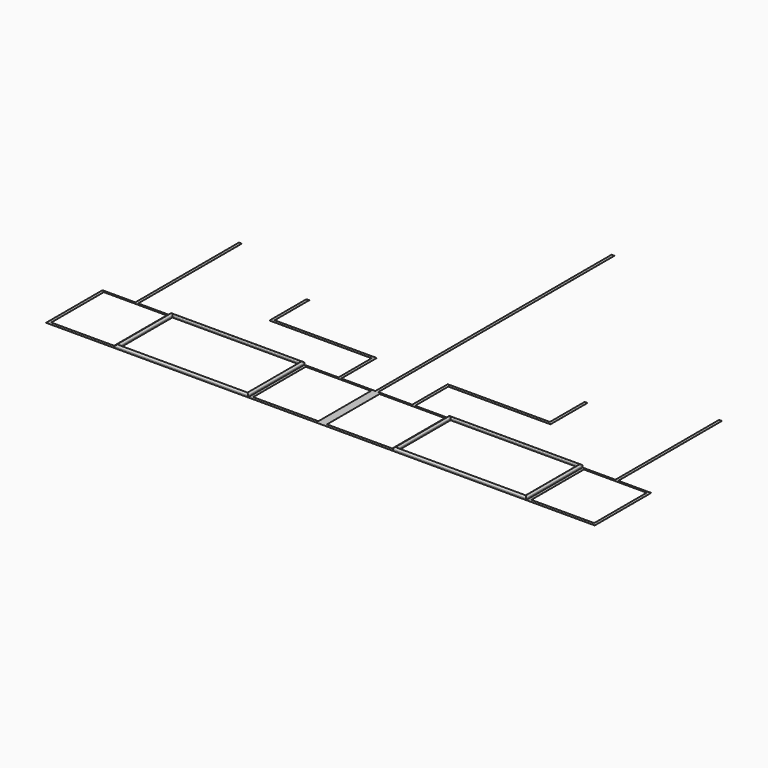
from build123d import *

# Parameters (mm, degrees)
F0_W         = 9.525
F0_H         = 457.2
F1_DEPTH     = 0.254
F0_W_2       = 19.05
F0_H_2       = 863.6
F2_DEPTH     = 19.05
F3_T1_DEPTH  = 936.625
F3_T3_DEPTH  = 517.525
F3_T5_DEPTH  = 850.9
F3_T7_DEPTH  = 438.15
F3_T13_DEPTH = 874.7125
F3_T17_DEPTH = 461.9625
F3_T24_DEPTH = 874.7125
F3_T28_DEPTH = 461.9625
F3_T35_DEPTH = 461.9625
F3_T39_DEPTH = 874.7125
F3_T46_DEPTH = 874.7125
F3_T50_DEPTH = 461.9625
F4_DEPTH     = 0.254
F5_DEPTH     = 19.05
F6_T3_DEPTH  = 517.525
F6_T6_DEPTH  = 936.625
F6_T9_DEPTH  = 517.525
F6_T12_DEPTH = 936.625
F6_T15_DEPTH = 850.9
F6_T18_DEPTH = 438.15
F6_T21_DEPTH = 850.9
F6_T24_DEPTH = 438.15
F6_T28_DEPTH = 874.7125
F6_T32_DEPTH = 461.9625
F6_T38_DEPTH = 874.7125
F6_T42_DEPTH = 461.9625
F6_T48_DEPTH = 461.9625
F6_T52_DEPTH = 874.7125
F6_T58_DEPTH = 874.7125
F6_T62_DEPTH = 461.9625


# Not quite as in the source:
# - a fillet or chamfer that OpenCascade refuses, or shapes differently, is made with other operations: its cross-section is extruded or revolved along the edge and cut away or added
# - a feature names something its author has since deleted; it is built from what else it names


with BuildPart() as f1:
    # F0 (on Top) → F1 (new body)
    with BuildSketch(Plane.XY):
        Polygon((0, -793.75), (0, 1187.45), (-9.525, 1187.45), (-9.525, -781.05), (-9.525, -793.75), align=None)
        with Locations((-4.7625, -1022.35)):
            Rectangle(F0_W, F0_H)
        Polygon((-9.525, -793.75), (-9.525, -781.05), (-28.575, -781.05), (-236.5375, -781.05), (-255.5875, -781.05), (-463.55, -781.05), (-482.6, -781.05), (-482.6, -793.75), (-482.6, -1250.95), (-9.525, -1250.95), align=None)
        Polygon((-28.575, -1231.9), (-463.55, -1231.9), (-463.55, -793.75), (-255.5875, -793.75), (-236.5375, -793.75), (-28.575, -793.75), align=None, mode=Mode.SUBTRACT)
        Polygon((-255.5875, -781.05), (-236.5375, -781.05), (-236.5375, -485.775), (-917.575, -485.775), (-917.575, -196.85), (-936.625, -196.85), (-936.625, -504.825), (-936.3493996177, -504.825), (-917.575, -504.825), (-255.5875, -504.825), align=None)
    extrude(amount=F1_DEPTH)

    # F0 (on Top) → F4 (join)
    with BuildSketch(Plane.XY):
        Polygon((9.525, -781.05), (9.525, -793.75), (9.525, -1250.95), (482.6, -1250.95), (482.6, -793.75), (482.6, -781.05), (463.55, -781.05), (255.5875, -781.05), (236.5375, -781.05), (28.575, -781.05), align=None)
        Polygon((28.575, -793.75), (236.5375, -793.75), (255.5875, -793.75), (463.55, -793.75), (463.55, -1231.9), (28.575, -1231.9), align=None, mode=Mode.SUBTRACT)
        with Locations((4.7625, -1022.35)):
            Rectangle(F0_W, F0_H)
        with Locations((-4.7625, -1022.35)):
            Rectangle(F0_W, F0_H)
        Polygon((0, -793.75), (0, 1187.45), (-9.525, 1187.45), (-9.525, -781.05), (-9.525, -793.75), align=None)
        Polygon((9.525, 1187.45), (0, 1187.45), (0, -793.75), (9.525, -793.75), (9.525, -781.05), align=None)
        Polygon((236.5375, -485.775), (236.5375, -781.05), (255.5875, -781.05), (255.5875, -504.825), (917.575, -504.825), (936.3493996177, -504.825), (936.625, -504.825), (936.625, -196.85), (917.575, -196.85), (917.575, -485.775), align=None)
    extrude(amount=F4_DEPTH)


with BuildPart() as f1b:
    # F0 (on Top) → F1, piece 2 (new body)
    with BuildSketch(Plane.XY):
        Polygon((-1809.75, -781.05), (-1828.8, -781.05), (-1828.8, -1250.95), (-1371.6, -1250.95), (-1371.6, -793.75), (-1371.6, -781.05), (-1390.65, -781.05), (-1590.675, -781.05), (-1609.725, -781.05), align=None)
        Polygon((-1809.75, -1231.9), (-1809.75, -793.75), (-1609.725, -793.75), (-1590.675, -793.75), (-1390.65, -793.75), (-1390.65, -1231.9), align=None, mode=Mode.SUBTRACT)
        with Locations((-1600.2, -349.25)):
            Rectangle(F0_W_2, F0_H_2)
    extrude(amount=F1_DEPTH)


with BuildPart() as f2:
    # F0 (on Top) → F2 (new body)
    with BuildSketch(Plane.XY):
        Polygon((-1371.6, -1250.95), (-482.6, -1250.95), (-482.6, -793.75), (-482.6, -781.05), (-501.65, -781.05), (-1352.55, -781.05), (-1371.6, -781.05), (-1371.6, -793.75), align=None)
        Polygon((-501.65, -1231.9), (-1352.55, -1231.9), (-1352.55, -793.75), (-927.1, -793.75), (-501.65, -793.75), align=None, mode=Mode.SUBTRACT)
    extrude(amount=F2_DEPTH)

    # F3: fillet of radius 9.525 on 8 edges, made by hand

    # F3_s2 → F3_t1 (cut)
    with BuildSketch(Plane.YZ.offset(-1395.4125)):
        with BuildLine():
            ThreePointArc((-1250.95, 9.525), (-1248.1601920908, 16.2601920908), (-1241.425, 19.05))
            Line((-1241.425, 19.05), (-1250.95, 19.05))
            Line((-1250.95, 19.05), (-1250.95, 9.525))
        make_face()
        with BuildLine():
            ThreePointArc((-790.575, 19.05), (-783.8398079092, 16.2601920908), (-781.05, 9.525))
            Line((-781.05, 9.525), (-781.05, 19.05))
            Line((-781.05, 19.05), (-790.575, 19.05))
        make_face()
    extrude(amount=F3_T1_DEPTH, mode=Mode.SUBTRACT)

    # F3_s4 → F3_t3 (cut)
    with BuildSketch(Plane.XZ.offset(757.2375)):
        with BuildLine():
            ThreePointArc((-492.125, 19.05), (-485.3898079092, 16.2601920908), (-482.6, 9.525))
            Line((-482.6, 9.525), (-482.6, 19.05))
            Line((-482.6, 19.05), (-492.125, 19.05))
        make_face()
        with BuildLine():
            ThreePointArc((-1362.075, 19.05), (-1368.8101920908, 16.2601920908), (-1371.6, 9.525))
            Line((-1371.6, 9.525), (-1371.6, 19.05))
            Line((-1371.6, 19.05), (-1362.075, 19.05))
        make_face()
    extrude(amount=F3_T3_DEPTH, mode=Mode.SUBTRACT)

    # F3_s6 → F3_t5 (cut)
    with BuildSketch(Plane.YZ.offset(-1352.55)):
        with BuildLine():
            ThreePointArc((-1241.425, 19.05), (-1234.6898079092, 16.2601920908), (-1231.9, 9.525))
            Line((-1231.9, 9.525), (-1231.9, 19.05))
            Line((-1231.9, 19.05), (-1241.425, 19.05))
        make_face()
        with BuildLine():
            ThreePointArc((-784.225, 19.05), (-790.9601920908, 16.2601920908), (-793.75, 9.525))
            Line((-793.75, 9.525), (-793.75, 19.05))
            Line((-793.75, 19.05), (-784.225, 19.05))
        make_face()
    extrude(amount=F3_T5_DEPTH, mode=Mode.SUBTRACT)

    # F3_s8 → F3_t7 (cut)
    with BuildSketch(Plane.XZ.offset(793.75)):
        with BuildLine():
            ThreePointArc((-1362.075, 19.05), (-1355.3398079092, 16.2601920908), (-1352.55, 9.525))
            Line((-1352.55, 9.525), (-1352.55, 19.05))
            Line((-1352.55, 19.05), (-1362.075, 19.05))
        make_face()
        with BuildLine():
            ThreePointArc((-492.125, 19.05), (-498.8601920908, 16.2601920908), (-501.65, 9.525))
            Line((-501.65, 9.525), (-501.65, 19.05))
            Line((-501.65, 19.05), (-492.125, 19.05))
        make_face()
    extrude(amount=F3_T7_DEPTH, mode=Mode.SUBTRACT)


with BuildPart() as f3_tool11:
    # F3_s12 → F3_t13 (new body)
    with BuildSketch(Plane.YZ.offset(-477.8375)):
        with BuildLine():
            ThreePointArc((-1241.425, 19.05), (-1234.6898079092, 16.2601920908), (-1231.9, 9.525))
            Line((-1231.9, 9.525), (-1231.9, 19.05))
            Line((-1231.9, 19.05), (-1241.425, 19.05))
        make_face()
    extrude(amount=-F3_T13_DEPTH)

    split(bisect_by=Plane.YZ.offset(-501.65), keep=Keep.TOP)


with BuildPart() as f3_tool15:
    # F3_s16 → F3_t17 (new body)
    with BuildSketch(Plane.XZ.offset(793.75)):
        with BuildLine():
            ThreePointArc((-492.125, 19.05), (-498.8601920908, 16.2601920908), (-501.65, 9.525))
            Line((-501.65, 9.525), (-501.65, 19.05))
            Line((-501.65, 19.05), (-492.125, 19.05))
        make_face()
    extrude(amount=F3_T17_DEPTH)

    split(bisect_by=Plane.XZ.offset(1231.9), keep=Keep.TOP)


with BuildPart() as f3_tool11_1:
    add(f3_tool11.part)

    # F3_t19: intersect F3_tool15
    add(f3_tool15.part, mode=Mode.INTERSECT)


with BuildPart() as f2_1:
    add(f2.part)

    # F3_t9: cut F3_tool11
    add(f3_tool11_1.part, mode=Mode.SUBTRACT)


with BuildPart() as f3_tool22:
    # F3_s23 → F3_t24 (new body)
    with BuildSketch(Plane.YZ.offset(-501.65)):
        with BuildLine():
            ThreePointArc((-1241.425, 19.05), (-1234.6898079092, 16.2601920908), (-1231.9, 9.525))
            Line((-1231.9, 9.525), (-1231.9, 19.05))
            Line((-1231.9, 19.05), (-1241.425, 19.05))
        make_face()
    extrude(amount=-F3_T24_DEPTH)

    split(bisect_by=Plane.YZ.offset(-1352.55), keep=Keep.BOTTOM)


with BuildPart() as f3_tool26:
    # F3_s27 → F3_t28 (new body)
    with BuildSketch(Plane.XZ.offset(1255.7125)):
        with BuildLine():
            ThreePointArc((-1362.075, 19.05), (-1355.3398079092, 16.2601920908), (-1352.55, 9.525))
            Line((-1352.55, 9.525), (-1352.55, 19.05))
            Line((-1352.55, 19.05), (-1362.075, 19.05))
        make_face()
    extrude(amount=-F3_T28_DEPTH)

    split(bisect_by=Plane.XZ.offset(1231.9), keep=Keep.TOP)


with BuildPart() as f3_tool22_1:
    add(f3_tool22.part)

    # F3_t30: intersect F3_tool26
    add(f3_tool26.part, mode=Mode.INTERSECT)


with BuildPart() as f2_2:
    add(f2_1.part)

    # F3_t20: cut F3_tool22
    add(f3_tool22_1.part, mode=Mode.SUBTRACT)


with BuildPart() as f3_tool33:
    # F3_s34 → F3_t35 (new body)
    with BuildSketch(Plane.XZ.offset(1231.9)):
        with BuildLine():
            ThreePointArc((-1362.075, 19.05), (-1355.3398079092, 16.2601920908), (-1352.55, 9.525))
            Line((-1352.55, 9.525), (-1352.55, 19.05))
            Line((-1352.55, 19.05), (-1362.075, 19.05))
        make_face()
    extrude(amount=-F3_T35_DEPTH)

    split(bisect_by=Plane.XZ.offset(793.75), keep=Keep.BOTTOM)


with BuildPart() as f3_tool37:
    # F3_s38 → F3_t39 (new body)
    with BuildSketch(Plane.YZ.offset(-501.65)):
        with BuildLine():
            ThreePointArc((-784.225, 19.05), (-790.9601920908, 16.2601920908), (-793.75, 9.525))
            Line((-793.75, 9.525), (-793.75, 19.05))
            Line((-793.75, 19.05), (-784.225, 19.05))
        make_face()
    extrude(amount=-F3_T39_DEPTH)

    split(bisect_by=Plane.YZ.offset(-1352.55), keep=Keep.BOTTOM)


with BuildPart() as f3_tool33_1:
    add(f3_tool33.part)

    # F3_t41: intersect F3_tool37
    add(f3_tool37.part, mode=Mode.INTERSECT)


with BuildPart() as f2_3:
    add(f2_2.part)

    # F3_t31: cut F3_tool33
    add(f3_tool33_1.part, mode=Mode.SUBTRACT)


with BuildPart() as f3_tool44:
    # F3_s45 → F3_t46 (new body)
    with BuildSketch(Plane.YZ.offset(-477.8375)):
        with BuildLine():
            ThreePointArc((-784.225, 19.05), (-790.9601920908, 16.2601920908), (-793.75, 9.525))
            Line((-793.75, 9.525), (-793.75, 19.05))
            Line((-793.75, 19.05), (-784.225, 19.05))
        make_face()
    extrude(amount=-F3_T46_DEPTH)

    split(bisect_by=Plane.YZ.offset(-501.65), keep=Keep.TOP)


with BuildPart() as f3_tool48:
    # F3_s49 → F3_t50 (new body)
    with BuildSketch(Plane.XZ.offset(769.9375)):
        with BuildLine():
            ThreePointArc((-492.125, 19.05), (-498.8601920908, 16.2601920908), (-501.65, 9.525))
            Line((-501.65, 9.525), (-501.65, 19.05))
            Line((-501.65, 19.05), (-492.125, 19.05))
        make_face()
    extrude(amount=F3_T50_DEPTH)

    split(bisect_by=Plane.XZ.offset(793.75), keep=Keep.BOTTOM)


with BuildPart() as f3_tool44_1:
    add(f3_tool44.part)

    # F3_t52: intersect F3_tool48
    add(f3_tool48.part, mode=Mode.INTERSECT)


with BuildPart() as f2_4:
    add(f2_3.part)

    # F3_t42: cut F3_tool44
    add(f3_tool44_1.part, mode=Mode.SUBTRACT)


with BuildPart() as f4:
    # F0 (on Top) → F4, piece 2 (new body)
    with BuildSketch(Plane.XY):
        with Locations((1600.2, -349.25)):
            Rectangle(F0_W_2, F0_H_2)
        Polygon((1828.8, -1250.95), (1828.8, -781.05), (1809.75, -781.05), (1609.725, -781.05), (1590.675, -781.05), (1390.65, -781.05), (1371.6, -781.05), (1371.6, -793.75), (1371.6, -1250.95), align=None)
        Polygon((1590.675, -793.75), (1609.725, -793.75), (1809.75, -793.75), (1809.75, -1231.9), (1390.65, -1231.9), (1390.65, -793.75), align=None, mode=Mode.SUBTRACT)
    extrude(amount=F4_DEPTH)


with BuildPart() as f5:
    # F0 (on Top) → F5 (new body)
    with BuildSketch(Plane.XY):
        Polygon((482.6, -793.75), (482.6, -1250.95), (1371.6, -1250.95), (1371.6, -793.75), (1371.6, -781.05), (1352.55, -781.05), (501.65, -781.05), (482.6, -781.05), align=None)
        Polygon((927.1, -793.75), (1352.55, -793.75), (1352.55, -1231.9), (501.65, -1231.9), (501.65, -793.75), align=None, mode=Mode.SUBTRACT)
    extrude(amount=F5_DEPTH)

    # F6: fillet of radius 9.525 on 8 edges, made by hand


with BuildPart() as f6_tool1:
    # F6_s2 → F6_t3 (new body)
    with BuildSketch(Plane.XZ.offset(1274.7625)):
        with BuildLine():
            ThreePointArc((482.6, 9.525), (485.3898079092, 16.2601920908), (492.125, 19.05))
            Line((492.125, 19.05), (482.6, 19.05))
            Line((482.6, 19.05), (482.6, 9.525))
        make_face()
    extrude(amount=-F6_T3_DEPTH)


with BuildPart() as f6_tool4:
    # F6_s5 → F6_t6 (new body)
    with BuildSketch(Plane.YZ.offset(458.7875)):
        with BuildLine():
            ThreePointArc((-1241.425, 19.05), (-1248.1601920908, 16.2601920908), (-1250.95, 9.525))
            Line((-1250.95, 9.525), (-1250.95, 19.05))
            Line((-1250.95, 19.05), (-1241.425, 19.05))
        make_face()
    extrude(amount=F6_T6_DEPTH)


with BuildPart() as f6_tool7:
    # F6_s8 → F6_t9 (new body)
    with BuildSketch(Plane.XZ.offset(757.2375)):
        with BuildLine():
            ThreePointArc((1362.075, 19.05), (1368.8101920908, 16.2601920908), (1371.6, 9.525))
            Line((1371.6, 9.525), (1371.6, 19.05))
            Line((1371.6, 19.05), (1362.075, 19.05))
        make_face()
    extrude(amount=F6_T9_DEPTH)


with BuildPart() as f6_tool10:
    # F6_s11 → F6_t12 (new body)
    with BuildSketch(Plane.YZ.offset(458.7875)):
        with BuildLine():
            ThreePointArc((-790.575, 19.05), (-783.8398079092, 16.2601920908), (-781.05, 9.525))
            Line((-781.05, 9.525), (-781.05, 19.05))
            Line((-781.05, 19.05), (-790.575, 19.05))
        make_face()
    extrude(amount=F6_T12_DEPTH)


with BuildPart() as f6_tool13:
    # F6_s14 → F6_t15 (new body)
    with BuildSketch(Plane.YZ.offset(1352.55)):
        with BuildLine():
            ThreePointArc((-784.225, 19.05), (-790.9601920908, 16.2601920908), (-793.75, 9.525))
            Line((-793.75, 9.525), (-793.75, 19.05))
            Line((-793.75, 19.05), (-784.225, 19.05))
        make_face()
    extrude(amount=-F6_T15_DEPTH)


with BuildPart() as f6_tool16:
    # F6_s17 → F6_t18 (new body)
    with BuildSketch(Plane.XZ.offset(793.75)):
        with BuildLine():
            ThreePointArc((1362.075, 19.05), (1355.3398079092, 16.2601920908), (1352.55, 9.525))
            Line((1352.55, 9.525), (1352.55, 19.05))
            Line((1352.55, 19.05), (1362.075, 19.05))
        make_face()
    extrude(amount=F6_T18_DEPTH)


with BuildPart() as f6_tool19:
    # F6_s20 → F6_t21 (new body)
    with BuildSketch(Plane.YZ.offset(1352.55)):
        with BuildLine():
            ThreePointArc((-1241.425, 19.05), (-1234.6898079092, 16.2601920908), (-1231.9, 9.525))
            Line((-1231.9, 9.525), (-1231.9, 19.05))
            Line((-1231.9, 19.05), (-1241.425, 19.05))
        make_face()
    extrude(amount=-F6_T21_DEPTH)


with BuildPart() as f6_tool22:
    # F6_s23 → F6_t24 (new body)
    with BuildSketch(Plane.XZ.offset(1231.9)):
        with BuildLine():
            ThreePointArc((492.125, 19.05), (498.8601920908, 16.2601920908), (501.65, 9.525))
            Line((501.65, 9.525), (501.65, 19.05))
            Line((501.65, 19.05), (492.125, 19.05))
        make_face()
    extrude(amount=-F6_T24_DEPTH)


with BuildPart() as f6_tool26:
    # F6_s27 → F6_t28 (new body)
    with BuildSketch(Plane.YZ.offset(1376.3625)):
        with BuildLine():
            ThreePointArc((-784.225, 19.05), (-790.9601920908, 16.2601920908), (-793.75, 9.525))
            Line((-793.75, 9.525), (-793.75, 19.05))
            Line((-793.75, 19.05), (-784.225, 19.05))
        make_face()
    extrude(amount=-F6_T28_DEPTH)

    split(bisect_by=Plane.YZ.offset(1352.55), keep=Keep.TOP)


with BuildPart() as f6_tool30:
    # F6_s31 → F6_t32 (new body)
    with BuildSketch(Plane.XZ.offset(769.9375)):
        with BuildLine():
            ThreePointArc((1362.075, 19.05), (1355.3398079092, 16.2601920908), (1352.55, 9.525))
            Line((1352.55, 9.525), (1352.55, 19.05))
            Line((1352.55, 19.05), (1362.075, 19.05))
        make_face()
    extrude(amount=F6_T32_DEPTH)

    split(bisect_by=Plane.XZ.offset(793.75), keep=Keep.BOTTOM)


with BuildPart() as f6_tool26_1:
    add(f6_tool26.part)

    # F6_t34: intersect F6_tool30
    add(f6_tool30.part, mode=Mode.INTERSECT)


with BuildPart() as f6_tool36:
    # F6_s37 → F6_t38 (new body)
    with BuildSketch(Plane.YZ.offset(1352.55)):
        with BuildLine():
            ThreePointArc((-784.225, 19.05), (-790.9601920908, 16.2601920908), (-793.75, 9.525))
            Line((-793.75, 9.525), (-793.75, 19.05))
            Line((-793.75, 19.05), (-784.225, 19.05))
        make_face()
    extrude(amount=-F6_T38_DEPTH)

    split(bisect_by=Plane.YZ.offset(501.65), keep=Keep.BOTTOM)


with BuildPart() as f6_tool40:
    # F6_s41 → F6_t42 (new body)
    with BuildSketch(Plane.XZ.offset(1231.9)):
        with BuildLine():
            ThreePointArc((492.125, 19.05), (498.8601920908, 16.2601920908), (501.65, 9.525))
            Line((501.65, 9.525), (501.65, 19.05))
            Line((501.65, 19.05), (492.125, 19.05))
        make_face()
    extrude(amount=-F6_T42_DEPTH)

    split(bisect_by=Plane.XZ.offset(793.75), keep=Keep.BOTTOM)


with BuildPart() as f6_tool36_1:
    add(f6_tool36.part)

    # F6_t44: intersect F6_tool40
    add(f6_tool40.part, mode=Mode.INTERSECT)


with BuildPart() as f6_tool46:
    # F6_s47 → F6_t48 (new body)
    with BuildSketch(Plane.XZ.offset(793.75)):
        with BuildLine():
            ThreePointArc((1362.075, 19.05), (1355.3398079092, 16.2601920908), (1352.55, 9.525))
            Line((1352.55, 9.525), (1352.55, 19.05))
            Line((1352.55, 19.05), (1362.075, 19.05))
        make_face()
    extrude(amount=F6_T48_DEPTH)

    split(bisect_by=Plane.XZ.offset(1231.9), keep=Keep.TOP)


with BuildPart() as f6_tool50:
    # F6_s51 → F6_t52 (new body)
    with BuildSketch(Plane.YZ.offset(1376.3625)):
        with BuildLine():
            ThreePointArc((-1241.425, 19.05), (-1234.6898079092, 16.2601920908), (-1231.9, 9.525))
            Line((-1231.9, 9.525), (-1231.9, 19.05))
            Line((-1231.9, 19.05), (-1241.425, 19.05))
        make_face()
    extrude(amount=-F6_T52_DEPTH)

    split(bisect_by=Plane.YZ.offset(1352.55), keep=Keep.TOP)


with BuildPart() as f6_tool46_1:
    add(f6_tool46.part)

    # F6_t54: intersect F6_tool50
    add(f6_tool50.part, mode=Mode.INTERSECT)


with BuildPart() as f6_tool56:
    # F6_s57 → F6_t58 (new body)
    with BuildSketch(Plane.YZ.offset(1352.55)):
        with BuildLine():
            ThreePointArc((-1241.425, 19.05), (-1234.6898079092, 16.2601920908), (-1231.9, 9.525))
            Line((-1231.9, 9.525), (-1231.9, 19.05))
            Line((-1231.9, 19.05), (-1241.425, 19.05))
        make_face()
    extrude(amount=-F6_T58_DEPTH)

    split(bisect_by=Plane.YZ.offset(501.65), keep=Keep.BOTTOM)


with BuildPart() as f6_tool60:
    # F6_s61 → F6_t62 (new body)
    with BuildSketch(Plane.XZ.offset(1255.7125)):
        with BuildLine():
            ThreePointArc((492.125, 19.05), (498.8601920908, 16.2601920908), (501.65, 9.525))
            Line((501.65, 9.525), (501.65, 19.05))
            Line((501.65, 19.05), (492.125, 19.05))
        make_face()
    extrude(amount=-F6_T62_DEPTH)

    split(bisect_by=Plane.XZ.offset(1231.9), keep=Keep.TOP)


with BuildPart() as f6_tool56_1:
    add(f6_tool56.part)

    # F6_t64: intersect F6_tool60
    add(f6_tool60.part, mode=Mode.INTERSECT)


with BuildPart() as f5_1:
    add(f5.part)

    # F6_t65: cut F6_tool1, F6_tool4, F6_tool7, F6_tool10, F6_tool13, F6_tool16, F6_tool19, F6_tool22, F6_tool26, F6_tool36, F6_tool46, F6_tool56
    add([f6_tool1.part, f6_tool4.part, f6_tool7.part, f6_tool10.part, f6_tool13.part, f6_tool16.part, f6_tool19.part, f6_tool22.part, f6_tool26_1.part, f6_tool36_1.part, f6_tool46_1.part, f6_tool56_1.part], mode=Mode.SUBTRACT)


solid = Compound([f1.part, f1b.part, f2_4.part, f4.part, f5_1.part])
